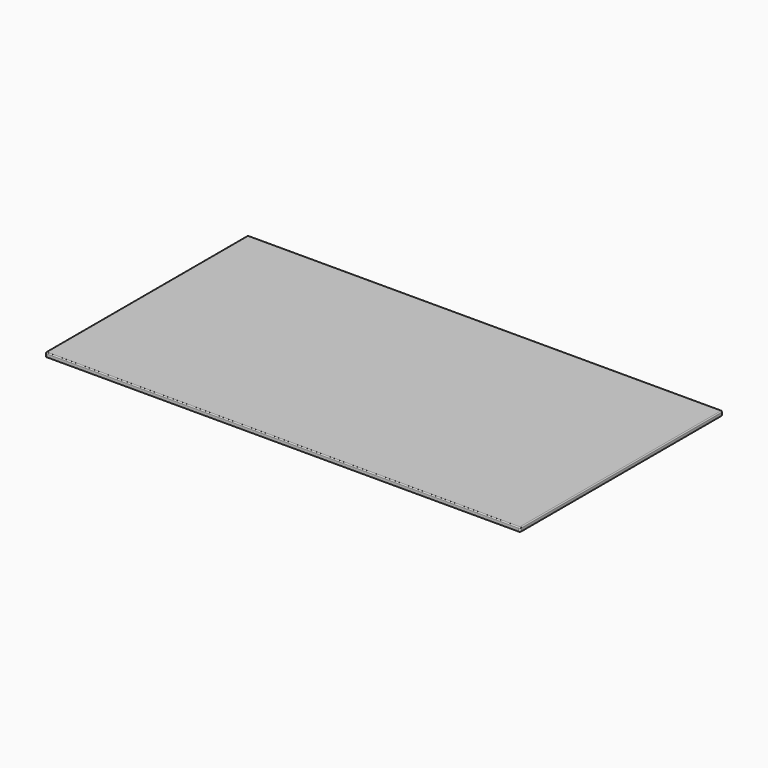
from build123d import *

# Parameters (mm, degrees)
F0_W         = 1500
F0_H         = 800
F1_DEPTH     = 25
F2_C1_SIZE2  = 21
F2_C1_SIZE   = 12.5
F2_C2_SIZE2  = 21
F2_C2_SIZE   = 12.5
F2_C3_SIZE2  = 12.5
F2_C3_SIZE   = 21
F2_C4_SIZE2  = 12.5
F2_C4_SIZE   = 21
F3_R         = 3
F4_T1_DEPTH  = 25
F4_T3_DEPTH  = 41.9202637387
F4_T5_DEPTH  = 41.9202637387
F4_T7_DEPTH  = 41.9202637387
F4_T9_DEPTH  = 41.9202637387
F4_T12_ANGLE = 90
F4_T14_ANGLE = 90
F4_T16_ANGLE = 90
F4_T18_ANGLE = 90


# Not quite as in the source:
# - a fillet or chamfer that OpenCascade refuses, or shapes differently, is made with other operations: its cross-section is extruded or revolved along the edge and cut away or added


with BuildPart() as f1:
    # F0 (on Top) → F1 (new body)
    with BuildSketch(Plane.XY):
        with Locations((-750, 400)):
            Rectangle(F0_W, F0_H)
    extrude(amount=F1_DEPTH)

    # F2: chamfer of 21 x 12.5 on 4 edges, made by hand

    # F2_c1
    f2_c1_edges = [f1.edges().sort_by_distance(p)[0] for p in [
        (-750, 0, 0),
    ]]
    f2_c1_side = f1.faces().sort_by_distance((-750, 0, 0.25))[0]
    chamfer(f2_c1_edges, length=F2_C1_SIZE, length2=F2_C1_SIZE2, reference=f2_c1_side)

    # F2_c2
    f2_c2_edges = [f1.edges().sort_by_distance(p)[0] for p in [
        (0, 410.5, 0),
    ]]
    f2_c2_side = f1.faces().sort_by_distance((0, 410.5, 0.25))[0]
    chamfer(f2_c2_edges, length=F2_C2_SIZE, length2=F2_C2_SIZE2, reference=f2_c2_side)

    # F2_c3
    f2_c3_edges = [f1.edges().sort_by_distance(p)[0] for p in [
        (-760.5, 800, 0),
    ]]
    f2_c3_side = f1.faces().sort_by_distance((-760.5, 799.75, 0))[0]
    chamfer(f2_c3_edges, length=F2_C3_SIZE, length2=F2_C3_SIZE2, reference=f2_c3_side)

    # F2_c4
    f2_c4_edges = [f1.edges().sort_by_distance(p)[0] for p in [
        (-1500, 400, 0),
    ]]
    f2_c4_side = f1.faces().sort_by_distance((-1499.75, 400, 0))[0]
    chamfer(f2_c4_edges, length=F2_C4_SIZE, length2=F2_C4_SIZE2, reference=f2_c4_side)

    # F3
    f3_edges = [f1.edges().sort_by_distance(p)[0] for p in [
        (-750, 0, 25),
        (0, 400, 25),
        (-750, 800, 25),
        (-1500, 400, 25),
    ]]
    fillet(f3_edges, radius=F3_R)

    # F4: fillet of radius 5 on 8 edges, made by hand

    # F4_s2 → F4_t1 (cut)
    with BuildSketch(Plane.XY):
        with BuildLine():
            ThreePointArc((-1500, 5), (-1498.5355339059, 1.4644660941), (-1495, 0))
            Line((-1495, 0), (-1500, 0))
            Line((-1500, 0), (-1500, 5))
        make_face()
        with BuildLine():
            ThreePointArc((-1495, 800), (-1498.5355339059, 798.5355339059), (-1500, 795))
            Line((-1500, 795), (-1500, 800))
            Line((-1500, 800), (-1495, 800))
        make_face()
        with BuildLine():
            ThreePointArc((-5, 800), (-1.4644660941, 798.5355339059), (0, 795))
            Line((0, 795), (0, 800))
            Line((0, 800), (-5, 800))
        make_face()
        with BuildLine():
            ThreePointArc((0, 5), (-1.4644660941, 1.4644660941), (-5, 0))
            Line((-5, 0), (0, 0))
            Line((0, 0), (0, 5))
        make_face()
    extrude(amount=F4_T1_DEPTH, mode=Mode.SUBTRACT)

    # F4_s4 → F4_t3 (cut)
    with BuildSketch(Plane(origin=(-616.1297856971, -616.1297856971, 366.7439200578), x_dir=(0.7071067812, -0.7071067812, 0), z_dir=(-0.6517309188, -0.6517309188, 0.3879350707))):
        with BuildLine():
            ThreePointArc((-1062.4685403084, -399.2446653395), (-1060.6601717798, -399.5831416331), (-1058.8518032513, -399.2446653395))
            Line((-1058.8518032513, -399.2446653395), (-1060.6601717798, -399.9461949124))
            Line((-1060.6601717798, -399.9461949124), (-1062.4685403084, -399.2446653395))
        make_face()
    extrude(amount=F4_T3_DEPTH, mode=Mode.SUBTRACT)

    # F4_s6 → F4_t5 (cut)
    with BuildSketch(Plane(origin=(-955.9323380689, 955.9323380689, 569.0073440886), x_dir=(-0.7071067812, -0.7071067812, 0), z_dir=(-0.6517309188, 0.6517309188, 0.3879350707))):
        with BuildLine():
            ThreePointArc((493.166378302, -618.693880655), (494.9747468306, -619.0323569486), (496.7831153591, -618.693880655))
            Line((496.7831153591, -618.693880655), (494.9747468306, -619.3954102279))
            Line((494.9747468306, -619.3954102279), (493.166378302, -618.693880655))
        make_face()
    extrude(amount=F4_T5_DEPTH, mode=Mode.SUBTRACT)

    # F4_s8 → F4_t7 (cut)
    with BuildSketch(Plane(origin=(318.8025523718, 318.8025523718, 189.7634240308), x_dir=(-0.7071067812, 0.7071067812, 0), z_dir=(0.6517309188, 0.6517309188, 0.3879350707))):
        with BuildLine():
            ThreePointArc((567.4937934778, -207.2266019385), (565.6854249492, -207.5650782321), (563.8770564207, -207.2266019385))
            Line((563.8770564207, -207.2266019385), (565.6854249492, -207.9281315114))
            Line((565.6854249492, -207.9281315114), (567.4937934778, -207.2266019385))
        make_face()
    extrude(amount=F4_T7_DEPTH, mode=Mode.SUBTRACT)

    # F4_s10 → F4_t9 (cut)
    with BuildSketch(Plane(origin=(6.320732001, -6.320732001, 3.7623404768), x_dir=(-0.7071067812, -0.7071067812, 0), z_dir=(-0.6517309188, 0.6517309188, -0.3879350707))):
        with BuildLine():
            ThreePointArc((-1.8083685285, 12.222613377), (0, 11.8841370834), (1.8083685285, 12.222613377))
            Line((1.8083685285, 12.222613377), (0, 11.5210838041))
            Line((0, 11.5210838041), (-1.8083685285, 12.222613377))
        make_face()
    extrude(amount=F4_T9_DEPTH, mode=Mode.SUBTRACT)

    # F4_s11 → F4_t12 (revolve, cut)
    with BuildSketch(Plane.YZ.offset(-5)):
        with BuildLine():
            ThreePointArc((3, 25), (0.8786796564, 24.1213203436), (0, 22))
            Line((0, 22), (0, 25))
            Line((0, 25), (3, 25))
        make_face()
    revolve(axis=Axis((-5, 5, 25), (0, 0, 1)), revolution_arc=F4_T12_ANGLE, mode=Mode.SUBTRACT)

    # F4_s13 → F4_t14 (revolve, cut)
    with BuildSketch(Plane.XZ.offset(-795)):
        with BuildLine():
            ThreePointArc((-3, 25), (-0.8786796564, 24.1213203436), (0, 22))
            Line((0, 22), (0, 25))
            Line((0, 25), (-3, 25))
        make_face()
    revolve(axis=Axis((-5, 795, 25), (0, 0, 1)), revolution_arc=F4_T14_ANGLE, mode=Mode.SUBTRACT)

    # F4_s15 → F4_t16 (revolve, cut)
    with BuildSketch(Plane.YZ.offset(-1495)):
        with BuildLine():
            ThreePointArc((797, 25), (799.1213203436, 24.1213203436), (800, 22))
            Line((800, 22), (800, 25))
            Line((800, 25), (797, 25))
        make_face()
    revolve(axis=Axis((-1495, 795, 25), (0, 0, 1)), revolution_arc=F4_T16_ANGLE, mode=Mode.SUBTRACT)

    # F4_s17 → F4_t18 (revolve, cut)
    with BuildSketch(Plane.XZ.offset(-5)):
        with BuildLine():
            ThreePointArc((-1497, 25), (-1499.1213203436, 24.1213203436), (-1500, 22))
            Line((-1500, 22), (-1500, 25))
            Line((-1500, 25), (-1497, 25))
        make_face()
    revolve(axis=Axis((-1495, 5, 25), (0, 0, 1)), revolution_arc=F4_T18_ANGLE, mode=Mode.SUBTRACT)


solid = f1.part
